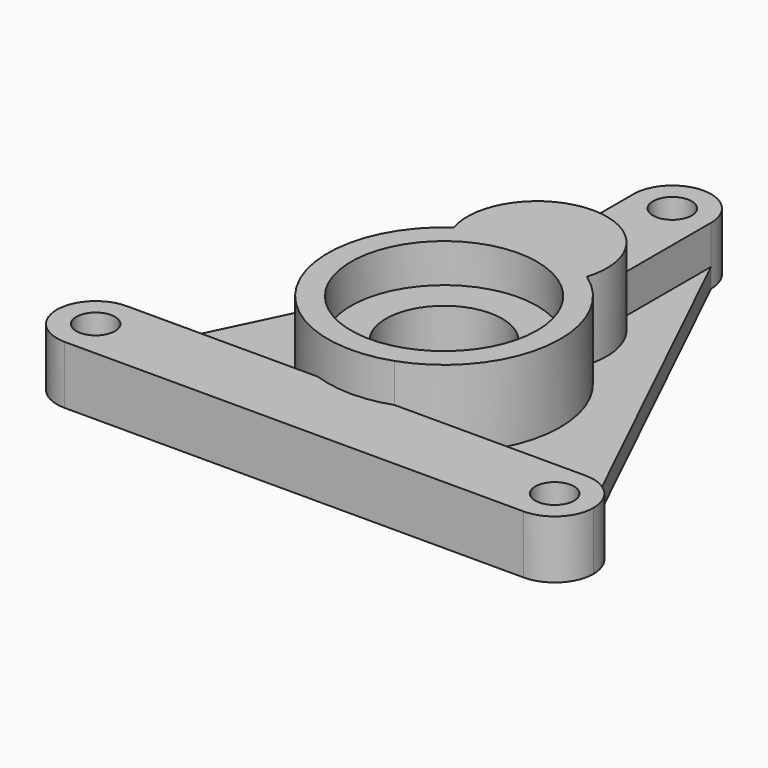
from build123d import *

# Parameters (mm, degrees)
F0_R     = 18
F0_R_2   = 15
F1_DEPTH = 25
F0_R_3   = 5
F2_DEPTH = 15
F3_DEPTH = 5
F4_R     = 24
F5_DEPTH = 10
F6_R     = 18
F7_DEPTH = 4
F8_DEPTH = 25


# Not quite as in the source:
# - a feature of the source that left no trace in its solid (it failed there, or was rolled back) is left out


with BuildPart() as f1:
    # F0 (on Top) → F1 (new body)
    with BuildSketch(Plane.XY):
        with BuildLine():
            ThreePointArc((11, 30), (10.9532905474, 28.9873667079), (10.8135588756, 27.9833333333))
            ThreePointArc((10.8135588756, 27.9833333333), (14.0941228696, 26.4831210498), (17.1709056255, 24.6))
            ThreePointArc((17.1709056255, 24.6), (16.9783517429, 35.9779237278), (10, 44.9666295471))
            ThreePointArc((10, 44.9666295471), (0, 48), (-10, 44.9666295471))
            ThreePointArc((-10, 44.9666295471), (-16.9783517429, 35.9779237278), (-17.1709056255, 24.6))
            ThreePointArc((-17.1709056255, 24.6), (-14.0941228696, 26.4831210498), (-10.8135588756, 27.9833333333))
            ThreePointArc((-10.8135588756, 27.9833333333), (-1.0126332921, 40.9532905474), (11, 30))
        make_face()
        with BuildLine():
            ThreePointArc((-7.9285699986, 28.9333333333), (0, 30), (7.9285699986, 28.9333333333))
            ThreePointArc((7.9285699986, 28.9333333333), (7.9821225244, 29.4654721656), (8, 30))
            ThreePointArc((8, 30), (-0.5345278344, 37.9821225244), (-7.9285699986, 28.9333333333))
        make_face()
        with BuildLine():
            ThreePointArc((7.9285699986, 28.9333333333), (9.3830951015, 28.4948684208), (10.8135588756, 27.9833333333))
            ThreePointArc((10.8135588756, 27.9833333333), (10.9532905474, 28.9873667079), (11, 30))
            ThreePointArc((11, 30), (-1.0126332921, 40.9532905474), (-10.8135588756, 27.9833333333))
            ThreePointArc((-10.8135588756, 27.9833333333), (-9.3830951015, 28.4948684208), (-7.9285699986, 28.9333333333))
            ThreePointArc((-7.9285699986, 28.9333333333), (-0.5345278344, 37.9821225244), (8, 30))
            ThreePointArc((8, 30), (7.9821225244, 29.4654721656), (7.9285699986, 28.9333333333))
        make_face()
        with BuildLine():
            ThreePointArc((8.1236109924, 22.5833333333), (19.6337294447, 13.8027775499), (24, 0))
            ThreePointArc((24, 0), (-13.8027775499, -19.6337294447), (-8.1236109924, 22.5833333333))
            ThreePointArc((-8.1236109924, 22.5833333333), (-9.8460195334, 25.0953186293), (-10.8135588756, 27.9833333333))
            ThreePointArc((-10.8135588756, 27.9833333333), (-14.0941228696, 26.4831210498), (-17.1709056255, 24.6))
            ThreePointArc((-17.1709056255, 24.6), (-29.7210146782, -4.0818239184), (-9.9032129289, -28.3183045694))
            ThreePointArc((-9.9032129289, -28.3183045694), (0, -30), (9.9032129289, -28.3183045694))
            ThreePointArc((9.9032129289, -28.3183045694), (24.4652446122, -17.3623675248), (30, 0))
            ThreePointArc((30, 0), (26.6000673755, 13.8721453142), (17.1709056255, 24.6))
            ThreePointArc((17.1709056255, 24.6), (14.0941228696, 26.4831210498), (10.8135588756, 27.9833333333))
            ThreePointArc((10.8135588756, 27.9833333333), (9.8460195334, 25.0953186293), (8.1236109924, 22.5833333333))
        make_face()
        with BuildLine():
            ThreePointArc((-8.1236109924, 22.5833333333), (-13.8027775499, -19.6337294447), (24, 0))
            ThreePointArc((24, 0), (19.6337294447, 13.8027775499), (8.1236109924, 22.5833333333))
            ThreePointArc((8.1236109924, 22.5833333333), (0, 19), (-8.1236109924, 22.5833333333))
        make_face()
        Circle(F0_R, mode=Mode.SUBTRACT)
        Circle(F0_R)
        Circle(F0_R_2, mode=Mode.SUBTRACT)
        Circle(F0_R_2)
        with BuildLine():
            ThreePointArc((-8.1236109924, 22.5833333333), (0, 19), (8.1236109924, 22.5833333333))
            ThreePointArc((8.1236109924, 22.5833333333), (6.4342628666, 23.1214242936), (4.7098006563, 23.5333333333))
            ThreePointArc((4.7098006563, 23.5333333333), (0, 22), (-4.7098006563, 23.5333333333))
            ThreePointArc((-4.7098006563, 23.5333333333), (-6.4342628666, 23.1214242936), (-8.1236109924, 22.5833333333))
        make_face()
        with BuildLine():
            ThreePointArc((4.7098006563, 23.5333333333), (6.4342628666, 23.1214242936), (8.1236109924, 22.5833333333))
            ThreePointArc((8.1236109924, 22.5833333333), (9.8460195334, 25.0953186293), (10.8135588756, 27.9833333333))
            ThreePointArc((10.8135588756, 27.9833333333), (9.3830951015, 28.4948684208), (7.9285699986, 28.9333333333))
            ThreePointArc((7.9285699986, 28.9333333333), (6.8718340494, 25.9039168957), (4.7098006563, 23.5333333333))
        make_face()
        with BuildLine():
            ThreePointArc((-10.8135588756, 27.9833333333), (-9.8460195334, 25.0953186293), (-8.1236109924, 22.5833333333))
            ThreePointArc((-8.1236109924, 22.5833333333), (-6.4342628666, 23.1214242936), (-4.7098006563, 23.5333333333))
            ThreePointArc((-4.7098006563, 23.5333333333), (-6.8718340494, 25.9039168957), (-7.9285699986, 28.9333333333))
            ThreePointArc((-7.9285699986, 28.9333333333), (-9.3830951015, 28.4948684208), (-10.8135588756, 27.9833333333))
        make_face()
        with BuildLine():
            ThreePointArc((-4.7098006563, 23.5333333333), (0, 24), (4.7098006563, 23.5333333333))
            ThreePointArc((4.7098006563, 23.5333333333), (6.8718340494, 25.9039168957), (7.9285699986, 28.9333333333))
            ThreePointArc((7.9285699986, 28.9333333333), (0, 30), (-7.9285699986, 28.9333333333))
            ThreePointArc((-7.9285699986, 28.9333333333), (-6.8718340494, 25.9039168957), (-4.7098006563, 23.5333333333))
        make_face()
        with BuildLine():
            ThreePointArc((-4.7098006563, 23.5333333333), (0, 22), (4.7098006563, 23.5333333333))
            ThreePointArc((4.7098006563, 23.5333333333), (0, 24), (-4.7098006563, 23.5333333333))
        make_face()
    extrude(amount=F1_DEPTH)

    # F0 (on Top) → F2 (join)
    with BuildSketch(Plane.XY):
        with BuildLine():
            ThreePointArc((9.9032129289, -28.3183045694), (0, -30), (-9.9032129289, -28.3183045694))
            Line((-9.9032129289, -28.3183045694), (-59.1904185712, -28.3183045694))
            ThreePointArc((-59.1904185712, -28.3183045694), (-52.1193507594, -31.2472367575), (-49.1904185712, -38.3183045694))
            ThreePointArc((-49.1904185712, -38.3183045694), (-52.1193507594, -45.3893723813), (-59.1904185712, -48.3183045694))
            Line((-59.1904185712, -48.3183045694), (0, -48.3183045694))
            Line((0, -48.3183045694), (59.1904185712, -48.3183045694))
            ThreePointArc((59.1904185712, -48.3183045694), (49.1904185712, -38.3183045694), (59.1904185712, -28.3183045694))
            Line((59.1904185712, -28.3183045694), (9.9032129289, -28.3183045694))
        make_face()
        with BuildLine():
            ThreePointArc((-49.1904185712, -38.3183045694), (-52.1193507594, -31.2472367575), (-59.1904185712, -28.3183045694))
            ThreePointArc((-59.1904185712, -28.3183045694), (-69.1904185712, -38.3183045694), (-59.1904185712, -48.3183045694))
            ThreePointArc((-59.1904185712, -48.3183045694), (-52.1193507594, -45.3893723813), (-49.1904185712, -38.3183045694))
        make_face()
        with Locations((-59.1904185712, -38.3183045694)):
            Circle(F0_R_3, mode=Mode.SUBTRACT)
        with BuildLine():
            ThreePointArc((69.1904185712, -38.3183045694), (66.2614863831, -31.2472367575), (59.1904185712, -28.3183045694))
            ThreePointArc((59.1904185712, -28.3183045694), (49.1904185712, -38.3183045694), (59.1904185712, -48.3183045694))
            ThreePointArc((59.1904185712, -48.3183045694), (66.2614863831, -45.3893723813), (69.1904185712, -38.3183045694))
        make_face()
        with Locations((59.1904185712, -38.3183045694)):
            Circle(F0_R_3, mode=Mode.SUBTRACT)
        with BuildLine():
            ThreePointArc((-10, 44.9666295471), (0, 48), (10, 44.9666295471))
            Line((10, 44.9666295471), (10, 73.5846459866))
            ThreePointArc((10, 73.5846459866), (0, 63.5846459866), (-10, 73.5846459866))
            Line((-10, 73.5846459866), (-10, 44.9666295471))
        make_face()
        with BuildLine():
            ThreePointArc((-10, 73.5846459866), (0, 63.5846459866), (10, 73.5846459866))
            ThreePointArc((10, 73.5846459866), (0, 83.5846459866), (-10, 73.5846459866))
        make_face()
        with Locations((0, 73.5846459866)):
            Circle(F0_R_3, mode=Mode.SUBTRACT)
    extrude(amount=F2_DEPTH)

    # F0 (on Top) → F3 (join)
    with BuildSketch(Plane.XY):
        with BuildLine():
            ThreePointArc((-9.9032129289, -28.3183045694), (-29.7210146782, -4.0818239184), (-17.1709056255, 24.6))
            ThreePointArc((-17.1709056255, 24.6), (-16.9783517429, 35.9779237278), (-10, 44.9666295471))
            Line((-10, 44.9666295471), (-10, 73.5846459866))
            Line((-10, 73.5846459866), (-59.1904185712, -28.3183045694))
            Line((-59.1904185712, -28.3183045694), (-9.9032129289, -28.3183045694))
        make_face()
        with BuildLine():
            ThreePointArc((10, 44.9666295471), (16.9783517429, 35.9779237278), (17.1709056255, 24.6))
            ThreePointArc((17.1709056255, 24.6), (26.6000673755, 13.8721453142), (30, 0))
            ThreePointArc((30, 0), (24.4652446122, -17.3623675248), (9.9032129289, -28.3183045694))
            Line((9.9032129289, -28.3183045694), (59.1904185712, -28.3183045694))
            Line((59.1904185712, -28.3183045694), (10, 73.5846459866))
            Line((10, 73.5846459866), (10, 44.9666295471))
        make_face()
    extrude(amount=F3_DEPTH)

    # F4 (on face) → F5 (cut)
    with BuildSketch(Plane.XY.offset(25)):
        Circle(F4_R)
    extrude(amount=-F5_DEPTH, mode=Mode.SUBTRACT)

    # F6 (on face) + F0 (on Top) → F7 (cut)
    with BuildSketch(Plane.XY):
        with BuildLine():
            ThreePointArc((10.8135588756, 27.9833333333), (9.8460195334, 25.0953186293), (8.1236109924, 22.5833333333))
            ThreePointArc((8.1236109924, 22.5833333333), (0, -24), (-8.1236109924, 22.5833333333))
            ThreePointArc((-8.1236109924, 22.5833333333), (-9.8460195334, 25.0953186293), (-10.8135588756, 27.9833333333))
            ThreePointArc((-10.8135588756, 27.9833333333), (-14.0941228696, 26.4831210498), (-17.1709056255, 24.6))
            ThreePointArc((-17.1709056255, 24.6), (-29.7210146782, -4.0818239184), (-9.9032129289, -28.3183045694))
            ThreePointArc((-9.9032129289, -28.3183045694), (0, -30), (9.9032129289, -28.3183045694))
            ThreePointArc((9.9032129289, -28.3183045694), (29.7210146782, -4.0818239184), (17.1709056255, 24.6))
            ThreePointArc((17.1709056255, 24.6), (14.0941228696, 26.4831210498), (10.8135588756, 27.9833333333))
        make_face()
        Circle(F6_R)
    with BuildSketch(Plane.XY):
        with BuildLine():
            ThreePointArc((-8.1236109924, 22.5833333333), (-13.8027775499, -19.6337294447), (24, 0))
            ThreePointArc((24, 0), (19.6337294447, 13.8027775499), (8.1236109924, 22.5833333333))
            ThreePointArc((8.1236109924, 22.5833333333), (0, 19), (-8.1236109924, 22.5833333333))
        make_face()
        Circle(F0_R, mode=Mode.SUBTRACT)
        Circle(F0_R)
        Circle(F0_R_2, mode=Mode.SUBTRACT)
        with BuildLine():
            ThreePointArc((-4.7098006563, 23.5333333333), (0, 24), (4.7098006563, 23.5333333333))
            ThreePointArc((4.7098006563, 23.5333333333), (6.8718340494, 25.9039168957), (7.9285699986, 28.9333333333))
            ThreePointArc((7.9285699986, 28.9333333333), (0, 30), (-7.9285699986, 28.9333333333))
            ThreePointArc((-7.9285699986, 28.9333333333), (-6.8718340494, 25.9039168957), (-4.7098006563, 23.5333333333))
        make_face()
        with BuildLine():
            ThreePointArc((-8.1236109924, 22.5833333333), (0, 19), (8.1236109924, 22.5833333333))
            ThreePointArc((8.1236109924, 22.5833333333), (6.4342628666, 23.1214242936), (4.7098006563, 23.5333333333))
            ThreePointArc((4.7098006563, 23.5333333333), (0, 22), (-4.7098006563, 23.5333333333))
            ThreePointArc((-4.7098006563, 23.5333333333), (-6.4342628666, 23.1214242936), (-8.1236109924, 22.5833333333))
        make_face()
        with BuildLine():
            ThreePointArc((-10.8135588756, 27.9833333333), (-9.8460195334, 25.0953186293), (-8.1236109924, 22.5833333333))
            ThreePointArc((-8.1236109924, 22.5833333333), (-6.4342628666, 23.1214242936), (-4.7098006563, 23.5333333333))
            ThreePointArc((-4.7098006563, 23.5333333333), (-6.8718340494, 25.9039168957), (-7.9285699986, 28.9333333333))
            ThreePointArc((-7.9285699986, 28.9333333333), (-9.3830951015, 28.4948684208), (-10.8135588756, 27.9833333333))
        make_face()
        with BuildLine():
            ThreePointArc((4.7098006563, 23.5333333333), (6.4342628666, 23.1214242936), (8.1236109924, 22.5833333333))
            ThreePointArc((8.1236109924, 22.5833333333), (9.8460195334, 25.0953186293), (10.8135588756, 27.9833333333))
            ThreePointArc((10.8135588756, 27.9833333333), (9.3830951015, 28.4948684208), (7.9285699986, 28.9333333333))
            ThreePointArc((7.9285699986, 28.9333333333), (6.8718340494, 25.9039168957), (4.7098006563, 23.5333333333))
        make_face()
        with BuildLine():
            ThreePointArc((-4.7098006563, 23.5333333333), (0, 22), (4.7098006563, 23.5333333333))
            ThreePointArc((4.7098006563, 23.5333333333), (0, 24), (-4.7098006563, 23.5333333333))
        make_face()
    extrude(amount=F7_DEPTH, mode=Mode.SUBTRACT)

    # F0 (on Top) → F8 (cut)
    with BuildSketch(Plane.XY):
        Circle(F0_R_2)
    extrude(amount=F8_DEPTH, mode=Mode.SUBTRACT)


solid = f1.part
